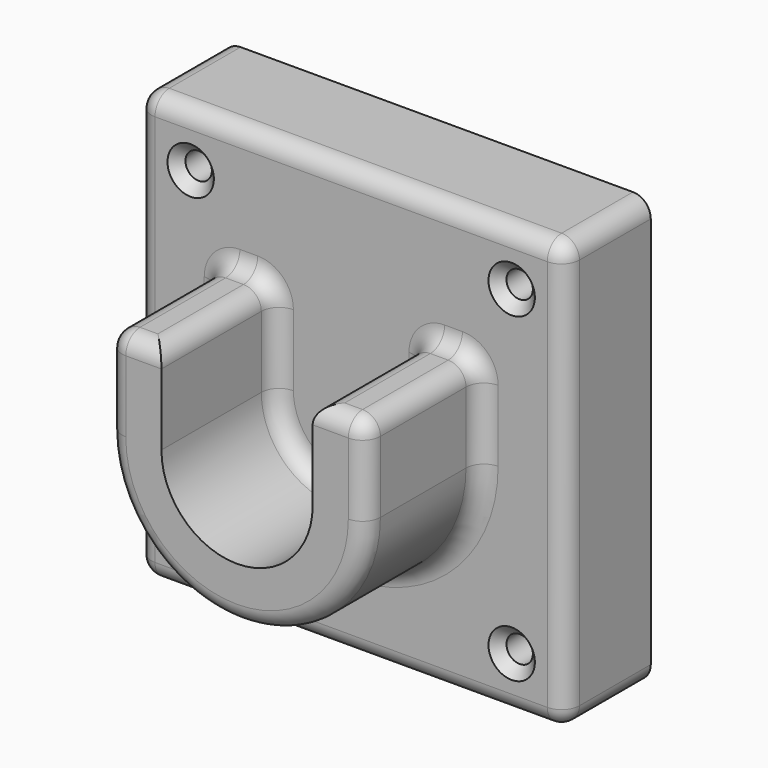
from build123d import *

# Parameters (mm, degrees)
F0_W           = 76.2
F0_H           = 76.2
F1_DEPTH       = 19.05
F3_DEPTH       = 25.4
F5_D           = 4.699
F5_CSINK_D     = 8.255
F5_CSINK_ANGLE = 90
F6_F1_R        = 3.175
F6_F2_R        = 3.175


with BuildPart() as f1:
    # F0 (on Front) → F1 (new body)
    with BuildSketch(Plane.XZ):
        Rectangle(F0_W, F0_H)
    extrude(amount=F1_DEPTH)

    # F2 (on face) → F3 (join)
    with BuildSketch(Plane.XZ.offset(19.05)):
        with BuildLine():
            ThreePointArc((13.462, 0), (0, -13.462), (-13.462, 0))
            Line((-13.462, 0), (-13.462, 15.875))
            Line((-13.462, 15.875), (-22.987, 15.875))
            Line((-22.987, 15.875), (-22.987, 0))
            ThreePointArc((-22.987, 0), (0, -22.987), (22.987, 0))
            Line((22.987, 0), (22.987, 15.875))
            Line((22.987, 15.875), (13.462, 15.875))
            Line((13.462, 15.875), (13.462, 0))
        make_face()
    extrude(amount=F3_DEPTH)

    # F5 (through all)
    with Locations(Plane.XZ.offset(19.05)):
        with Locations((-28.575, 28.575), (28.575, 28.575), (28.575, -28.575), (-28.575, -28.575)):
            CounterSinkHole(F5_D / 2, F5_CSINK_D / 2, counter_sink_angle=F5_CSINK_ANGLE)

    # F6: fillet of radius 3.175 on 23 edges, made by hand

    # F6_f1
    f6_f1_edges = [f1.edges().sort_by_distance(p)[0] for p in [
        (-38.1, -19.05, 0),
        (0, -19.05, 38.1),
        (38.1, -19.05, 0),
        (0, -19.05, -38.1),
        (0, -44.45, -22.987),
        (38.1, -9.525, -38.1),
        (38.1, -9.525, 38.1),
        (-38.1, -9.525, 38.1),
        (-38.1, -9.525, -38.1),
        (-13.462, -31.75, 15.875),
        (13.462, -31.75, 15.875),
        (22.987, -31.75, 15.875),
        (-22.987, -31.75, 15.875),
        (-18.2245, -44.45, 15.875),
        (18.2245, -44.45, 15.875),
        (22.987, -44.45, 7.9375),
        (-22.987, -44.45, 7.9375),
    ]]
    fillet(f6_f1_edges, radius=F6_F1_R)

    # F6_f2
    f6_f2_edges = [f1.edges().sort_by_distance(p)[0] for p in [
        (0, -19.05, -22.987),
        (0, -19.05, -13.462),
        (13.462, -19.05, 6.35),
        (-13.462, -19.05, 6.35),
        (22.987, -19.05, 6.35),
        (-22.987, -19.05, 6.35),
        (-22.0570640303, -19.05, 14.9450640303),
        (22.0570640303, -19.05, 14.9450640303),
        (-14.3919359697, -19.05, 14.9450640303),
        (14.3919359697, -19.05, 14.9450640303),
    ]]
    fillet(f6_f2_edges, radius=F6_F2_R)


solid = f1.part
